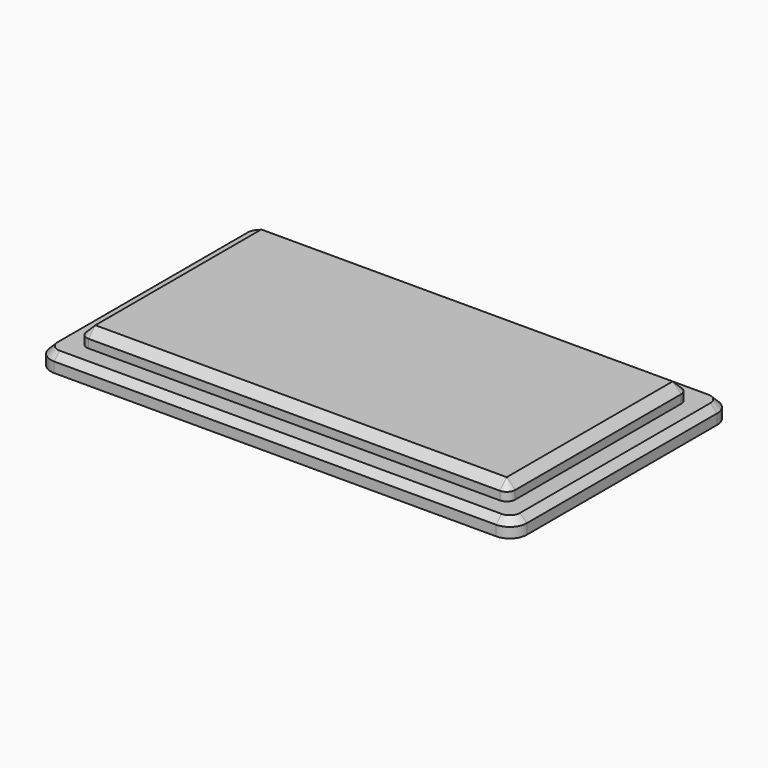
from build123d import *

# Parameters (mm, degrees)
F1_DEPTH = 12.7
F2_SIZE  = 5.08
F4_DEPTH = 12.7
F5_SIZE  = 6.34999


# Not quite as in the source:
# - a fillet or chamfer is up to 0.001 mm smaller than in the source, because OpenCascade refuses the exact size


with BuildPart() as f1:
    # F0 (on Top) → F1 (new body)
    with BuildSketch(Plane.XY):
        with BuildLine():
            Line((0, 190.5), (0, 12.7))
            ThreePointArc((0, 12.7), (3.7197438789, 3.7197438789), (12.7, 0))
            Line((12.7, 0), (342.9, 0))
            ThreePointArc((342.9, 0), (351.8802561211, 3.7197438789), (355.6, 12.7))
            Line((355.6, 12.7), (355.6, 190.5))
            ThreePointArc((355.6, 190.5), (351.8802561211, 199.4802561211), (342.9, 203.2))
            Line((342.9, 203.2), (12.7, 203.2))
            ThreePointArc((12.7, 203.2), (3.7197438789, 199.4802561211), (0, 190.5))
        make_face()
    extrude(amount=F1_DEPTH)

    # F2
    f2_edges = [f1.edges().sort_by_distance(p)[0] for p in [
        (0, 101.6, 12.7),
    ]]
    chamfer(f2_edges, length=F2_SIZE)

    # F3 (on face) → F4 (join)
    with BuildSketch(Plane.XY.offset(12.7)):
        with BuildLine():
            Line((17.78, 179.07), (17.78, 101.6))
            Line((17.78, 101.6), (17.78, 24.13))
            ThreePointArc((17.78, 24.13), (19.6398719395, 19.6398719395), (24.13, 17.78))
            Line((24.13, 17.78), (177.8, 17.78))
            Line((177.8, 17.78), (331.47, 17.78))
            ThreePointArc((331.47, 17.78), (335.9601280605, 19.6398719395), (337.82, 24.13))
            Line((337.82, 24.13), (337.82, 101.6))
            Line((337.82, 101.6), (337.82, 179.07))
            ThreePointArc((337.82, 179.07), (335.9601280605, 183.5601280605), (331.47, 185.42))
            Line((331.47, 185.42), (177.8, 185.42))
            Line((177.8, 185.42), (24.13, 185.42))
            ThreePointArc((24.13, 185.42), (19.6398719395, 183.5601280605), (17.78, 179.07))
        make_face()
    extrude(amount=F4_DEPTH)

    # F5 (size 6.35 in the source; OpenCascade refuses exactly that, so slightly less here)
    f5_edges = [f1.edges().sort_by_distance(p)[0] for p in [
        (177.8, 17.78, 25.4),
    ]]
    chamfer(f5_edges, length=F5_SIZE)


solid = f1.part
